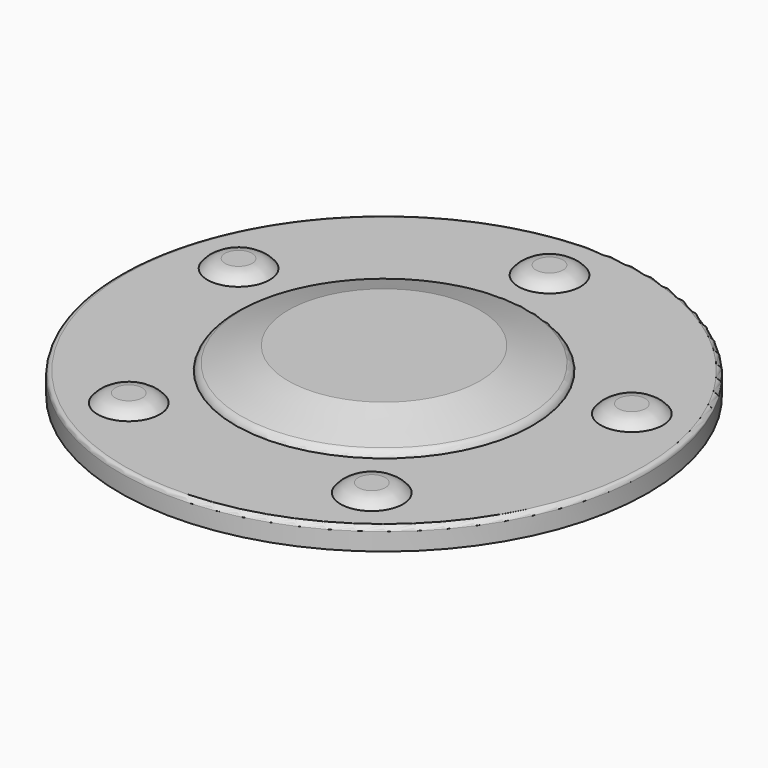
from build123d import *

# Parameters (mm, degrees)
F0_R     = 60
F1_DEPTH = 5
F2_R     = 1
F3_R     = 7.0850530083
F4_DEPTH = 2
F6_R     = 33.800823702
F7_DEPTH = 5
F8_SIZE2 = 4
F8_SIZE  = 12


# Not quite as in the source:
# - a fillet or chamfer that OpenCascade refuses, or shapes differently, is made with other operations: its cross-section is extruded or revolved along the edge and cut away or added
# - a feature names something its author has since deleted; it is built from what else it names


with BuildPart() as f1:
    # F0 (on Top) → F1 (new body)
    with BuildSketch(Plane.XY):
        Circle(F0_R)
    extrude(amount=F1_DEPTH)

    # F2
    f2_edges = [f1.edges().sort_by_distance(p)[0] for p in [
        (-60, 0, 5),
    ]]
    fillet(f2_edges, radius=F2_R)

    # F3 (on face) → F4 (join)
    with BuildSketch(Plane.XY.offset(5)):
        with Locations((0, 47)):
            Circle(F3_R)
        with Locations((-44.6996562659, 14.5237987356)):
            Circle(F3_R)
        with Locations((-27.6259068577, -38.0237987356)):
            Circle(F3_R)
        with Locations((27.6259068577, -38.0237987356)):
            Circle(F3_R)
        with Locations((44.6996562659, 14.5237987356)):
            Circle(F3_R)
    extrude(amount=F4_DEPTH)

    # F5: fillet of radius 5 on 5 edges, made by hand

    # F5_s1 → F5_t2 (revolve, cut)
    with BuildSketch(Plane.XZ.offset(-47)):
        with BuildLine():
            ThreePointArc((7.0850530083, 5), (5.3211209858, 6.472135955), (3.0850530083, 7))
            Line((3.0850530083, 7), (7.0850530083, 7))
            Line((7.0850530083, 7), (7.0850530083, 5))
        make_face()
    revolve(axis=Axis((0, 47, 7), (0, 0, 1)), mode=Mode.SUBTRACT)

    # F5_s3 → F5_t4 (revolve, cut)
    with BuildSketch(Plane.XZ.offset(-14.5237987356)):
        with BuildLine():
            ThreePointArc((51.7847092742, 5), (50.0207772517, 6.472135955), (47.7847092742, 7))
            Line((47.7847092742, 7), (51.7847092742, 7))
            Line((51.7847092742, 7), (51.7847092742, 5))
        make_face()
    revolve(axis=Axis((44.6996562659, 14.5237987356, 7), (0, 0, 1)), mode=Mode.SUBTRACT)

    # F5_s5 → F5_t6 (revolve, cut)
    with BuildSketch(Plane.XZ.offset(38.0237987356)):
        with BuildLine():
            ThreePointArc((34.7109598661, 5), (32.9470278436, 6.472135955), (30.7109598661, 7))
            Line((30.7109598661, 7), (34.7109598661, 7))
            Line((34.7109598661, 7), (34.7109598661, 5))
        make_face()
    revolve(axis=Axis((27.6259068577, -38.0237987356, 7), (0, 0, 1)), mode=Mode.SUBTRACT)

    # F5_s7 → F5_t8 (revolve, cut)
    with BuildSketch(Plane.XZ.offset(38.0237987356)):
        with BuildLine():
            ThreePointArc((-20.5408538494, 5), (-22.3047858719, 6.472135955), (-24.5408538494, 7))
            Line((-24.5408538494, 7), (-20.5408538494, 7))
            Line((-20.5408538494, 7), (-20.5408538494, 5))
        make_face()
    revolve(axis=Axis((-27.6259068577, -38.0237987356, 7), (0, 0, 1)), mode=Mode.SUBTRACT)

    # F5_s9 → F5_t10 (revolve, cut)
    with BuildSketch(Plane.XZ.offset(-14.5237987356)):
        with BuildLine():
            ThreePointArc((-37.6146032575, 5), (-39.37853528, 6.472135955), (-41.6146032575, 7))
            Line((-41.6146032575, 7), (-37.6146032575, 7))
            Line((-37.6146032575, 7), (-37.6146032575, 5))
        make_face()
    revolve(axis=Axis((-44.6996562659, 14.5237987356, 7), (0, 0, 1)), mode=Mode.SUBTRACT)

    # F6 (on face) → F7 (join)
    with BuildSketch(Plane.XY.offset(5)):
        Circle(F6_R)
    extrude(amount=F7_DEPTH)

    # F8
    f8_edges = [f1.edges().sort_by_distance(p)[0] for p in [
        (-33.800824, 0, 10),
    ]]
    f8_side = f1.faces().sort_by_distance((0, 0, 10))[0]
    chamfer(f8_edges, length=F8_SIZE, length2=F8_SIZE2, reference=f8_side)

    # F9: fillet of radius 2 on 1 edges, made by hand

    # F9_s1 → F9_t2 (revolve, cut)
    with BuildSketch(Plane.XZ):
        with BuildLine():
            ThreePointArc((33.800823702, 5), (33.33069476, 5.8898153625), (32.486741959, 6.4380272477))
            Line((32.486741959, 6.4380272477), (33.800823702, 6))
            Line((33.800823702, 6), (33.800823702, 5))
        make_face()
    revolve(axis=Axis((0, 0, 6), (0, 0, 1)), mode=Mode.SUBTRACT)


solid = f1.part
